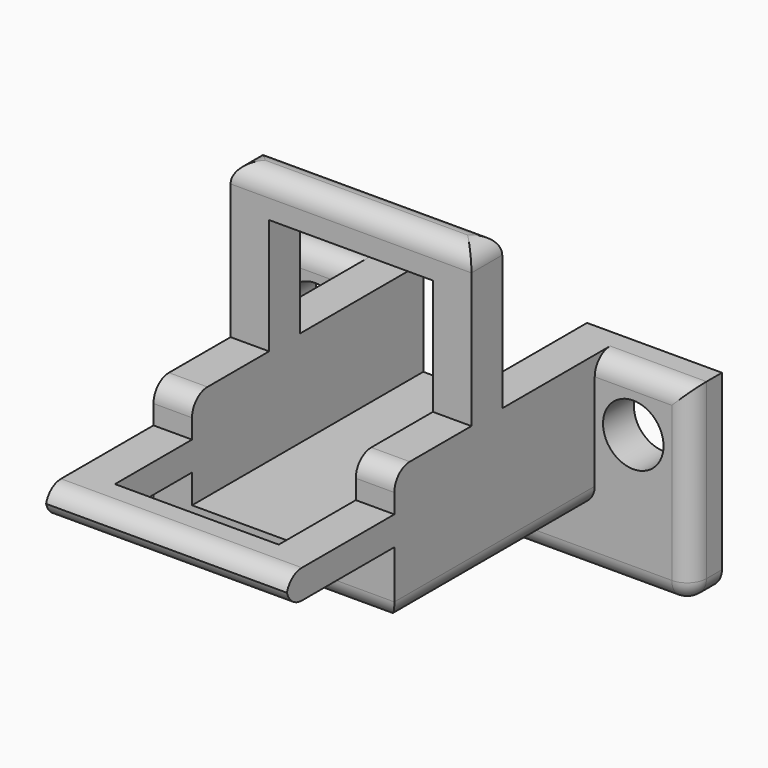
from build123d import *

# Parameters (mm, degrees)
F1_DEPTH      = 19.05
F0_R          = 1.9939
F2_DEPTH      = 2.54
F3_W          = 2.54
F3_H          = 1.905
F4_DEPTH      = 8.89
F5_W          = 2.54
F5_H          = 1.905
F6_DEPTH      = 11.43
F7_W          = 2.54
F7_H          = 2.54
F8_W          = 2.54
F8_H          = 2.54
F9_DEPTH      = 10.16
F10_W         = 2.54
F10_H         = 2.54
F11_DEPTH     = 11.43
F12_T1_DEPTH  = 9.525
F12_T3_DEPTH  = 14.605
F12_T5_DEPTH  = 26.035
F12_T7_DEPTH  = 9.525
F12_T9_DEPTH  = 4.445
F12_T11_DEPTH = 19.685
F12_T13_DEPTH = 22.225
F12_T15_DEPTH = 8.89
F12_T17_DEPTH = 8.89
F12_T19_DEPTH = 8.89
F12_S23_W     = 1.27
F12_S23_H     = 1.27
F12_T24_DEPTH = 1.27
F12_S29_W     = 1.27
F12_S29_H     = 1.27
F12_T30_DEPTH = 1.27


# Not quite as in the source:
# - a fillet or chamfer that OpenCascade refuses, or shapes differently, is made with other operations: its cross-section is extruded or revolved along the edge and cut away or added


with BuildPart() as f1:
    # F0 (on Front) → F1 (new body)
    with BuildSketch(Plane.XZ):
        Polygon((-23.2056408978, -6.35), (-23.2056408978, 0), (-25.7456408978, 0), (-25.7456408978, -8.89), (-9.8706408978, -8.89), (-9.8706408978, 0), (-12.4106408978, 0), (-12.4106408978, -6.35), align=None)
    extrude(amount=F1_DEPTH)

    # F0 (on Front) → F2 (join)
    with BuildSketch(Plane.XZ):
        Polygon((-25.7456408978, -8.89), (-25.7456408978, 0), (-32.0956408978, 0), (-32.0956408978, -12.7), (-3.5206408978, -12.7), (-3.5206408978, 0), (-9.8706408978, 0), (-9.8706408978, -8.89), align=None)
        with Locations((-28.2856408978, -3.81)):
            Circle(F0_R, mode=Mode.SUBTRACT)
        with Locations((-7.3306408978, -3.81)):
            Circle(F0_R, mode=Mode.SUBTRACT)
    extrude(amount=F2_DEPTH)

    # F3 (on face) → F4 (join)
    with BuildSketch(Plane.XZ.offset(19.05)):
        with Locations((-11.1406408978, -3.4925)):
            Rectangle(F3_W, F3_H)
        with Locations((-24.4756408978, -3.4925)):
            Rectangle(F3_W, F3_H)
    extrude(amount=F4_DEPTH)

    # F5 (on face) → F6 (join)
    with BuildSketch(Plane(origin=(-12.4106408978, 0, 0), x_dir=(0, -1, 0), z_dir=(-1, 0, 0))):
        with Locations((26.67, -3.4925)):
            Rectangle(F5_W, F5_H)
    extrude(amount=F6_DEPTH)

    # F7 (on face) + F8 (on face) → F9 (join)
    with BuildSketch(Plane.XY):
        with Locations((-24.4756408978, -11.43)):
            Rectangle(F7_W, F7_H)
    with BuildSketch(Plane.XY):
        with Locations((-11.1406408978, -11.43)):
            Rectangle(F8_W, F8_H)
    extrude(amount=F9_DEPTH)

    # F10 (on face) → F11 (join)
    with BuildSketch(Plane.YZ.offset(-23.2056408978)):
        with Locations((-11.43, 8.89)):
            Rectangle(F10_W, F10_H)
    extrude(amount=F11_DEPTH)

    # F12: fillet of radius 1.27 on 18 edges, made by hand

    # F12_s2 → F12_t1 (cut)
    with BuildSketch(Plane.YZ.offset(-35.2706408978)):
        with BuildLine():
            ThreePointArc((-1.27, 0), (-2.1680256121, -0.3719743879), (-2.54, -1.27))
            Line((-2.54, -1.27), (-2.54, 0))
            Line((-2.54, 0), (-1.27, 0))
        make_face()
    extrude(amount=F12_T1_DEPTH, mode=Mode.SUBTRACT)

    # F12_s4 → F12_t3 (cut)
    with BuildSketch(Plane.XY.offset(-11.43)):
        with BuildLine():
            ThreePointArc((-32.0956408978, -1.27), (-31.7236665099, -2.1680256121), (-30.8256408978, -2.54))
            Line((-30.8256408978, -2.54), (-32.0956408978, -2.54))
            Line((-32.0956408978, -2.54), (-32.0956408978, -1.27))
        make_face()
        with BuildLine():
            ThreePointArc((-3.5206408978, -1.27), (-3.8926152856, -2.1680256121), (-4.7906408978, -2.54))
            Line((-4.7906408978, -2.54), (-3.5206408978, -2.54))
            Line((-3.5206408978, -2.54), (-3.5206408978, -1.27))
        make_face()
    extrude(amount=F12_T3_DEPTH, mode=Mode.SUBTRACT)

    # F12_s6 → F12_t5 (cut)
    with BuildSketch(Plane.YZ.offset(-30.8256408978)):
        with BuildLine():
            ThreePointArc((-1.27, -12.7), (-2.1680256121, -12.3280256121), (-2.54, -11.43))
            Line((-2.54, -11.43), (-2.54, -12.7))
            Line((-2.54, -12.7), (-1.27, -12.7))
        make_face()
    extrude(amount=F12_T5_DEPTH, mode=Mode.SUBTRACT)

    # F12_s8 → F12_t7 (cut)
    with BuildSketch(Plane.YZ.offset(-9.8706408978)):
        with BuildLine():
            ThreePointArc((-1.27, 0), (-2.1680256121, -0.3719743879), (-2.54, -1.27))
            Line((-2.54, -1.27), (-2.54, 0))
            Line((-2.54, 0), (-1.27, 0))
        make_face()
    extrude(amount=F12_T7_DEPTH, mode=Mode.SUBTRACT)

    # F12_s10 → F12_t9 (cut)
    with BuildSketch(Plane.XZ.offset(-3.175)):
        with BuildLine():
            ThreePointArc((-4.7906408978, -12.7), (-3.8926152856, -12.3280256121), (-3.5206408978, -11.43))
            Line((-3.5206408978, -11.43), (-3.5206408978, -12.7))
            Line((-3.5206408978, -12.7), (-4.7906408978, -12.7))
        make_face()
        with BuildLine():
            ThreePointArc((-32.0956408978, -11.43), (-31.7236665099, -12.3280256121), (-30.8256408978, -12.7))
            Line((-30.8256408978, -12.7), (-32.0956408978, -12.7))
            Line((-32.0956408978, -12.7), (-32.0956408978, -11.43))
        make_face()
    extrude(amount=F12_T9_DEPTH, mode=Mode.SUBTRACT)

    # F12_s12 → F12_t11 (cut)
    with BuildSketch(Plane.XZ.offset(2.54)):
        with BuildLine():
            ThreePointArc((-9.8706408978, -7.62), (-10.2426152856, -8.5180256121), (-11.1406408978, -8.89))
            Line((-11.1406408978, -8.89), (-9.8706408978, -8.89))
            Line((-9.8706408978, -8.89), (-9.8706408978, -7.62))
        make_face()
        with BuildLine():
            ThreePointArc((-25.7456408978, -7.62), (-25.3736665099, -8.5180256121), (-24.4756408978, -8.89))
            Line((-24.4756408978, -8.89), (-25.7456408978, -8.89))
            Line((-25.7456408978, -8.89), (-25.7456408978, -7.62))
        make_face()
    extrude(amount=F12_T11_DEPTH, mode=Mode.SUBTRACT)

    # F12_s14 → F12_t13 (cut)
    with BuildSketch(Plane.YZ.offset(-28.9206408978)):
        with BuildLine():
            ThreePointArc((-26.67, -2.54), (-27.5680256121, -2.9119743879), (-27.94, -3.81))
            Line((-27.94, -3.81), (-27.94, -2.54))
            Line((-27.94, -2.54), (-26.67, -2.54))
        make_face()
        with BuildLine():
            ThreePointArc((-19.05, -7.62), (-18.6780256121, -8.5180256121), (-17.78, -8.89))
            Line((-17.78, -8.89), (-19.05, -8.89))
            Line((-19.05, -8.89), (-19.05, -7.62))
        make_face()
        with BuildLine():
            ThreePointArc((-27.94, -3.175), (-27.5680256121, -4.0730256121), (-26.67, -4.445))
            Line((-26.67, -4.445), (-27.94, -4.445))
            Line((-27.94, -4.445), (-27.94, -3.175))
        make_face()
        with BuildLine():
            ThreePointArc((-11.43, 10.16), (-12.3280256121, 9.7880256121), (-12.7, 8.89))
            Line((-12.7, 8.89), (-12.7, 10.16))
            Line((-12.7, 10.16), (-11.43, 10.16))
        make_face()
        with BuildLine():
            ThreePointArc((-10.16, 8.89), (-10.5319743879, 9.7880256121), (-11.43, 10.16))
            Line((-11.43, 10.16), (-10.16, 10.16))
            Line((-10.16, 10.16), (-10.16, 8.89))
        make_face()
    extrude(amount=F12_T13_DEPTH, mode=Mode.SUBTRACT)

    # F12_s16 → F12_t15 (cut)
    with BuildSketch(Plane.YZ.offset(-28.9206408978)):
        with BuildLine():
            ThreePointArc((-19.05, -1.27), (-18.6780256121, -0.3719743879), (-17.78, 0))
            Line((-17.78, 0), (-19.05, 0))
            Line((-19.05, 0), (-19.05, -1.27))
        make_face()
    extrude(amount=F12_T15_DEPTH, mode=Mode.SUBTRACT)

    # F12_s18 → F12_t17 (cut)
    with BuildSketch(Plane.YZ.offset(-15.5856408978)):
        with BuildLine():
            ThreePointArc((-17.78, 0), (-18.6780256121, -0.3719743879), (-19.05, -1.27))
            Line((-19.05, -1.27), (-19.05, 0))
            Line((-19.05, 0), (-17.78, 0))
        make_face()
    extrude(amount=F12_T17_DEPTH, mode=Mode.SUBTRACT)

    # F12_s20 → F12_t19 (cut)
    with BuildSketch(Plane.XZ.offset(6.985)):
        with BuildLine():
            ThreePointArc((-25.7456408978, 8.89), (-25.3736665099, 9.7880256121), (-24.4756408978, 10.16))
            Line((-24.4756408978, 10.16), (-25.7456408978, 10.16))
            Line((-25.7456408978, 10.16), (-25.7456408978, 8.89))
        make_face()
        with BuildLine():
            ThreePointArc((-9.8706408978, 8.89), (-10.2426152856, 9.7880256121), (-11.1406408978, 10.16))
            Line((-11.1406408978, 10.16), (-9.8706408978, 10.16))
            Line((-9.8706408978, 10.16), (-9.8706408978, 8.89))
        make_face()
    extrude(amount=F12_T19_DEPTH, mode=Mode.SUBTRACT)


with BuildPart() as f12_tool22:
    # F12_s23 → F12_t24 (new body)
    with BuildSketch(Plane.YZ.offset(-30.8256408978)):
        with Locations((-1.905, -12.065)):
            Rectangle(F12_S23_W, F12_S23_H)
    extrude(amount=-F12_T24_DEPTH)

    # F12_s25 → F12_t26 (revolve, cut)
    with BuildSketch(Plane(origin=(-30.8256408978, -1.27, -11.43), x_dir=(0, 0.7071067812, 0.7071067812), z_dir=(0, -0.7071067812, 0.7071067812))):
        with BuildLine():
            ThreePointArc((0, -1.27), (1.27, 0), (0, 1.27))
            Line((0, 1.27), (0, -1.27))
        make_face()
    revolve(axis=Axis((-30.8256408978, -1.27, -11.43), (-1, 0, 0)), mode=Mode.SUBTRACT)


with BuildPart() as f1_1:
    add(f1.part)

    # F12_t21: cut F12_tool22
    add(f12_tool22.part, mode=Mode.SUBTRACT)


with BuildPart() as f12_tool28:
    # F12_s29 → F12_t30 (new body)
    with BuildSketch(Plane.YZ.offset(-4.7906408978)):
        with Locations((-1.905, -12.065)):
            Rectangle(F12_S29_W, F12_S29_H)
    extrude(amount=F12_T30_DEPTH)

    # F12_s31 → F12_t32 (revolve, cut)
    with BuildSketch(Plane(origin=(-4.7906408978, -1.27, -11.43), x_dir=(0, 0.7071067812, 0.7071067812), z_dir=(0, 0.7071067812, -0.7071067812))):
        with BuildLine():
            ThreePointArc((0, -1.27), (1.27, 0), (0, 1.27))
            Line((0, 1.27), (0, -1.27))
        make_face()
    revolve(axis=Axis((-4.7906408978, -1.27, -11.43), (1, 0, 0)), mode=Mode.SUBTRACT)


with BuildPart() as f1_2:
    add(f1_1.part)

    # F12_t27: cut F12_tool28
    add(f12_tool28.part, mode=Mode.SUBTRACT)


solid = f1_2.part
